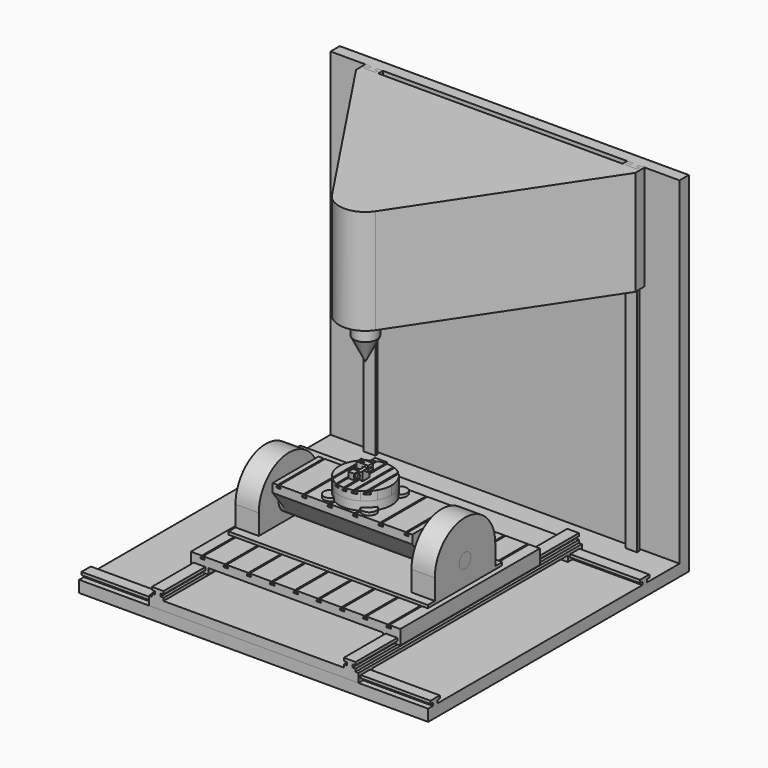
from build123d import *

# Parameters (mm, degrees)
F0_W           = 25.4
F0_H           = 12.7
F1_DEPTH       = 762
F3_DEPTH       = 457.2
F5_DEPTH       = 609.6
F7_DEPTH       = 381
F9_DEPTH       = 609.601
F9_DEPTH_BACK  = 609.601
F10_W          = 869.95
F10_H          = 12.7
F11_DEPTH      = 203.2
F14_DEPTH      = 101.6
F15_DEPTH      = 101.6
F16_R          = 31.75
F17_DEPTH      = 762.001
F17_DEPTH_BACK = 762.001
F18_R          = 31.75
F19_DEPTH      = 434.975
F19_DEPTH_BACK = 434.975
F20_DEPTH      = 333.375
F20_DEPTH_BACK = 333.375
F18_W          = 249.8384077759
F18_H          = 38.1
F21_DEPTH      = 304.8
F23_DEPTH      = 609.601
F23_DEPTH_BACK = 609.601
F25_DEPTH      = 12.7
F26_DEPTH      = 38.1
F27_DEPTH      = 38.1
F29_DEPTH      = 609.601
F29_DEPTH_BACK = 609.601
F30_DEPTH      = 152.4
F31_W          = 1524
F31_H          = 1524
F32_DEPTH      = 50.8
F34_DEPTH      = 1473.2
F36_DEPTH      = 457.2
F38_DEPTH      = 457.2
F39_R          = 50.8
F40_DEPTH      = 76.2
F44_DEPTH      = 38.1
F45_R          = 4.7625
F46_DEPTH      = 101.6
F47_W          = 19.05
F47_H          = 25.4
F48_DEPTH      = 25.4
F50_DEPTH      = 844.551
F51_R          = 4.7625
F52_DEPTH      = 101.6
F53_W          = 20.7483425409
F53_H          = 29.6389577031
F54_DEPTH      = 1035.051
F55_W          = 25.4
F55_H          = 25.4
F55_R          = 4.7625
F56_DEPTH      = 25.4
F57_R          = 7.9375
F58_DEPTH      = 9.525
F60_DEPTH      = 488.951


with BuildPart() as f1:
    # F0 (on Right) → F1 (new body, symmetric)
    with BuildSketch(Plane.YZ):
        Polygon((-558.8, -12.7), (-584.2, -12.7), (-609.6, -12.7), (-609.6, -63.5), (609.6, -63.5), (609.6, -12.7), (584.2, -12.7), (558.8, -12.7), align=None)
        Polygon((-596.9, 12.7), (-596.9, 0), (-584.2, 0), (-558.8, 0), (-546.1, 0), (-546.1, 12.7), align=None)
        with Locations((571.5, -6.35)):
            Rectangle(F0_W, F0_H)
        Polygon((546.1, 0), (558.8, 0), (584.2, 0), (596.9, 0), (596.9, 12.7), (546.1, 12.7), align=None)
        with Locations((-571.5, -6.35)):
            Rectangle(F0_W, F0_H)
    extrude(amount=F1_DEPTH, both=True)

    # F30 (add): a face of the model
    f30_faces = [f1.faces().sort_by_distance(p)[0] for p in [
        (0, 609.6, -38.1),
    ]]
    extrude(f30_faces, amount=F30_DEPTH)

    # F31 (on face) → F32 (join)
    with BuildSketch(Plane(origin=(0, 762, 0), x_dir=(-1, 0, 0), z_dir=(0, 1, 0))):
        with Locations((0, 698.5)):
            Rectangle(F31_W, F31_H)
    extrude(amount=F32_DEPTH)

    # F33 (on face) → F34 (join, through all)
    with BuildSketch(Plane.XY.offset(1460.5)):
        Polygon((584.2, 749.3), (584.2, 762), (558.8, 762), (558.8, 749.3), (546.1, 749.3), (546.1, 736.6), (596.9, 736.6), (596.9, 749.3), align=None)
        Polygon((-584.2, 762), (-584.2, 749.3), (-596.9, 749.3), (-596.9, 736.6), (-546.1, 736.6), (-546.1, 749.3), (-558.8, 749.3), (-558.8, 762), align=None)
    extrude(amount=-F34_DEPTH)


with BuildPart() as f3:
    # F2 (on Right) → F3 (new body, symmetric)
    with BuildSketch(Plane.YZ):
        Polygon((-609.6, 25.4), (-609.6, -12.7), (-584.2, -12.7), (-584.2, 0), (-596.9, 0), (-596.9, 12.7), (-546.1, 12.7), (-546.1, 0), (-558.8, 0), (-558.8, -12.7), (-533.4, -12.7), (-533.4, 12.7), (533.4, 12.7), (533.4, -12.7), (558.8, -12.7), (558.8, 0), (546.1, 0), (546.1, 12.7), (596.9, 12.7), (596.9, 0), (584.2, 0), (584.2, -12.7), (609.6, -12.7), (609.6, 25.4), align=None)
    extrude(amount=F3_DEPTH, both=True)

    # F4 (on Front) → F5 (join, symmetric)
    with BuildSketch(Plane.XZ):
        Polygon((-444.5, 38.1), (-444.5, 25.4), (-393.7, 25.4), (-393.7, 38.1), (-406.4, 38.1), (-406.4, 50.8), (-393.7, 50.8), (-393.7, 63.5), (-444.5, 63.5), (-444.5, 50.8), (-431.8, 50.8), (-431.8, 38.1), align=None)
        Polygon((393.7, 63.5), (393.7, 50.8), (406.4, 50.8), (406.4, 38.1), (393.7, 38.1), (393.7, 25.4), (444.5, 25.4), (444.5, 38.1), (431.8, 38.1), (431.8, 50.8), (444.5, 50.8), (444.5, 63.5), align=None)
    extrude(amount=F5_DEPTH, both=True)


with BuildPart() as f7:
    # F6 (on Front) → F7 (new body, symmetric)
    with BuildSketch(Plane.XZ):
        Polygon((-457.2, 38.1), (-431.8, 38.1), (-431.8, 50.8), (-444.5, 50.8), (-444.5, 63.5), (-393.7, 63.5), (-393.7, 50.8), (-406.4, 50.8), (-406.4, 38.1), (-381, 38.1), (-381, 63.5), (381, 63.5), (381, 38.1), (406.4, 38.1), (406.4, 50.8), (393.7, 50.8), (393.7, 63.5), (444.5, 63.5), (444.5, 50.8), (431.8, 50.8), (431.8, 38.1), (457.2, 38.1), (457.2, 101.6), (-457.2, 101.6), align=None)
    extrude(amount=F7_DEPTH, both=True)

    # F8 (on Front) → F9 (cut, two sides)
    with BuildSketch(Plane.XZ) as f9_sk:
        Polygon((-403.225, 101.6), (-409.575, 101.6), (-409.575, 95.25), (-415.925, 95.25), (-415.925, 88.9), (-396.875, 88.9), (-396.875, 95.25), (-403.225, 95.25), align=None)
        Polygon((-295.275, 95.25), (-301.625, 95.25), (-301.625, 101.6), (-307.975, 101.6), (-307.975, 95.25), (-314.325, 95.25), (-314.325, 88.9), (-295.275, 88.9), align=None)
        Polygon((-193.675, 95.25), (-200.025, 95.25), (-200.025, 101.6), (-206.375, 101.6), (-206.375, 95.25), (-212.725, 95.25), (-212.725, 88.9), (-193.675, 88.9), align=None)
        Polygon((-92.075, 95.25), (-98.425, 95.25), (-98.425, 101.6), (-104.775, 101.6), (-104.775, 95.25), (-111.125, 95.25), (-111.125, 88.9), (-92.075, 88.9), align=None)
        Polygon((9.525, 95.25), (3.175, 95.25), (3.175, 101.6), (-3.175, 101.6), (-3.175, 95.25), (-9.525, 95.25), (-9.525, 88.9), (9.525, 88.9), align=None)
        Polygon((111.125, 95.25), (104.775, 95.25), (104.775, 101.6), (98.425, 101.6), (98.425, 95.25), (92.075, 95.25), (92.075, 88.9), (111.125, 88.9), align=None)
        Polygon((212.725, 95.25), (206.375, 95.25), (206.375, 101.6), (200.025, 101.6), (200.025, 95.25), (193.675, 95.25), (193.675, 88.9), (212.725, 88.9), align=None)
        Polygon((314.325, 95.25), (307.975, 95.25), (307.975, 101.6), (301.625, 101.6), (301.625, 95.25), (295.275, 95.25), (295.275, 88.9), (314.325, 88.9), align=None)
        Polygon((415.925, 95.25), (409.575, 95.25), (409.575, 101.6), (403.225, 101.6), (403.225, 95.25), (396.875, 95.25), (396.875, 88.9), (415.925, 88.9), align=None)
    extrude(amount=-F9_DEPTH, mode=Mode.SUBTRACT)
    extrude(f9_sk.sketch, amount=F9_DEPTH_BACK, mode=Mode.SUBTRACT)


with BuildPart() as f11:
    # F10 (on Front) → F11 (new body, symmetric)
    with BuildSketch(Plane.XZ):
        with Locations((0, 107.95)):
            Rectangle(F10_W, F10_H)
    extrude(amount=F11_DEPTH, both=True)

    # F13 (on face) → F14 (join)
    with BuildSketch(Plane.YZ.offset(434.975)):
        with BuildLine():
            ThreePointArc((165.1, 203.2), (0, 368.3), (-165.1, 203.2))
            Line((-165.1, 203.2), (-165.1, 114.3))
            Line((-165.1, 114.3), (165.1, 114.3))
            Line((165.1, 114.3), (165.1, 203.2))
        make_face()
    extrude(amount=-F14_DEPTH)

    # F12 (on face) → F15 (join)
    with BuildSketch(Plane(origin=(-434.975, 0, 0), x_dir=(0, -1, 0), z_dir=(-1, 0, 0))):
        with BuildLine():
            Line((-165.1, 203.2), (-165.1, 114.3))
            Line((-165.1, 114.3), (165.1, 114.3))
            Line((165.1, 114.3), (165.1, 203.2))
            ThreePointArc((165.1, 203.2), (0, 368.3), (-165.1, 203.2))
        make_face()
    extrude(amount=-F15_DEPTH)

    # F16 (on Right) → F17 (cut, two sides)
    with BuildSketch(Plane.YZ) as f17_sk:
        with Locations((0, 203.2)):
            Circle(F16_R)
    extrude(amount=-F17_DEPTH, mode=Mode.SUBTRACT)
    extrude(f17_sk.sketch, amount=F17_DEPTH_BACK, mode=Mode.SUBTRACT)


with BuildPart() as f19:
    # F18 (on Right) → F19 (new body, two sides)
    with BuildSketch(Plane.YZ) as f19_sk:
        with Locations((0, 203.2)):
            Circle(F18_R)
    extrude(amount=-F19_DEPTH)
    extrude(f19_sk.sketch, amount=F19_DEPTH_BACK)

    # F18 (on Right) → F20 (join, two sides)
    with BuildSketch(Plane.YZ) as f20_sk:
        with BuildLine():
            ThreePointArc((-45.4898926883, 168.6053159689), (0, 146.05), (45.4898926883, 168.6053159689))
            ThreePointArc((45.4898926883, 168.6053159689), (54.1565779344, 184.946573844), (57.15, 203.2))
            ThreePointArc((57.15, 203.2), (-18.253426156, 257.3565779344), (-45.4898926883, 168.6053159689))
        make_face()
        with Locations((0, 203.2)):
            Circle(F18_R, mode=Mode.SUBTRACT)
    extrude(amount=F20_DEPTH)
    extrude(f20_sk.sketch, amount=-F20_DEPTH_BACK)

    # F18 (on Right) → F21 (join, symmetric)
    with BuildSketch(Plane.YZ):
        with BuildLine():
            Line((45.4898926883, 168.6053159689), (124.919203888, 273.05))
            Line((124.919203888, 273.05), (-124.919203888, 273.05))
            Line((-124.919203888, 273.05), (-45.4898926883, 168.6053159689))
            ThreePointArc((-45.4898926883, 168.6053159689), (-18.253426156, 257.3565779344), (57.15, 203.2))
            ThreePointArc((57.15, 203.2), (54.1565779344, 184.946573844), (45.4898926883, 168.6053159689))
        make_face()
        with Locations((0, 292.1)):
            Rectangle(F18_W, F18_H)
    extrude(amount=F21_DEPTH, both=True)

    # F22 (on Front) → F23 (cut, two sides)
    with BuildSketch(Plane.XZ) as f23_sk:
        Polygon((282.575, 304.8), (282.575, 311.15), (276.225, 311.15), (276.225, 304.8), (269.875, 304.8), (269.875, 298.45), (288.925, 298.45), (288.925, 304.8), align=None)
        Polygon((158.115, 304.8), (158.115, 298.45), (177.165, 298.45), (177.165, 304.8), (170.815, 304.8), (170.815, 311.15), (164.465, 311.15), (164.465, 304.8), align=None)
        Polygon((46.355, 304.8), (46.355, 298.45), (65.405, 298.45), (65.405, 304.8), (59.055, 304.8), (59.055, 311.15), (52.705, 311.15), (52.705, 304.8), align=None)
        Polygon((-65.405, 304.8), (-65.405, 298.45), (-46.355, 298.45), (-46.355, 304.8), (-52.705, 304.8), (-52.705, 311.15), (-59.055, 311.15), (-59.055, 304.8), align=None)
        Polygon((-177.165, 304.8), (-177.165, 298.45), (-158.115, 298.45), (-158.115, 304.8), (-164.465, 304.8), (-164.465, 311.15), (-170.815, 311.15), (-170.815, 304.8), align=None)
        Polygon((-288.925, 304.8), (-288.925, 298.45), (-269.875, 298.45), (-269.875, 304.8), (-276.225, 304.8), (-276.225, 311.15), (-282.575, 311.15), (-282.575, 304.8), align=None)
    extrude(amount=-F23_DEPTH, mode=Mode.SUBTRACT)
    extrude(f23_sk.sketch, amount=F23_DEPTH_BACK, mode=Mode.SUBTRACT)


with BuildPart() as f25:
    # F24 (on face) → F25 (new body)
    with BuildSketch(Plane.XY.offset(311.15)):
        with BuildLine():
            ThreePointArc((98.9867036526, -57.15), (110.4053219448, -29.5830168552), (114.3, 0))
            ThreePointArc((114.3, 0), (110.4053219448, 29.5830168552), (98.9867036526, 57.15))
            ThreePointArc((98.9867036526, 57.15), (80.8223050896, 80.8223050896), (57.15, 98.9867036526))
            ThreePointArc((57.15, 98.9867036526), (0, 114.3), (-57.15, 98.9867036526))
            ThreePointArc((-57.15, 98.9867036526), (-80.8223050896, 80.8223050896), (-98.9867036526, 57.15))
            ThreePointArc((-98.9867036526, 57.15), (-114.3, 0), (-98.9867036526, -57.15))
            ThreePointArc((-98.9867036526, -57.15), (-80.8223050896, -80.8223050896), (-57.15, -98.9867036526))
            ThreePointArc((-57.15, -98.9867036526), (0, -114.3), (57.15, -98.9867036526))
            ThreePointArc((57.15, -98.9867036526), (80.8223050896, -80.8223050896), (98.9867036526, -57.15))
        make_face()
        with BuildLine():
            ThreePointArc((57.15, 98.9867036526), (80.8223050896, 80.8223050896), (98.9867036526, 57.15))
            ThreePointArc((98.9867036526, 57.15), (105.3296786843, 105.3296786843), (57.15, 98.9867036526))
        make_face()
        with BuildLine():
            ThreePointArc((57.15, -98.9867036526), (105.3296786843, -105.3296786843), (98.9867036526, -57.15))
            ThreePointArc((98.9867036526, -57.15), (80.8223050896, -80.8223050896), (57.15, -98.9867036526))
        make_face()
        with BuildLine():
            ThreePointArc((-98.9867036526, 57.15), (-80.8223050896, 80.8223050896), (-57.15, 98.9867036526))
            ThreePointArc((-57.15, 98.9867036526), (-105.3296786843, 105.3296786843), (-98.9867036526, 57.15))
        make_face()
        with BuildLine():
            ThreePointArc((-98.9867036526, -57.15), (-105.3296786843, -105.3296786843), (-57.15, -98.9867036526))
            ThreePointArc((-57.15, -98.9867036526), (-80.8223050896, -80.8223050896), (-98.9867036526, -57.15))
        make_face()
    extrude(amount=F25_DEPTH)

    # F24 (on face) → F26 (join)
    with BuildSketch(Plane.XY.offset(311.15)):
        with BuildLine():
            ThreePointArc((98.9867036526, -57.15), (110.4053219448, -29.5830168552), (114.3, 0))
            ThreePointArc((114.3, 0), (110.4053219448, 29.5830168552), (98.9867036526, 57.15))
            ThreePointArc((98.9867036526, 57.15), (80.8223050896, 80.8223050896), (57.15, 98.9867036526))
            ThreePointArc((57.15, 98.9867036526), (0, 114.3), (-57.15, 98.9867036526))
            ThreePointArc((-57.15, 98.9867036526), (-58.1052206891, 98.4290268603), (-59.055, 97.8621324875))
            Line((-59.055, 97.8621324875), (-59.055, -97.8621324875))
            ThreePointArc((-59.055, -97.8621324875), (-58.1052206891, -98.4290268603), (-57.15, -98.9867036526))
            ThreePointArc((-57.15, -98.9867036526), (0, -114.3), (57.15, -98.9867036526))
            ThreePointArc((57.15, -98.9867036526), (80.8223050896, -80.8223050896), (98.9867036526, -57.15))
        make_face()
        with BuildLine():
            Line((-59.055, -97.8621324875), (-59.055, 97.8621324875))
            ThreePointArc((-59.055, 97.8621324875), (-81.6006400482, 80.0364013667), (-98.9867036526, 57.15))
            ThreePointArc((-98.9867036526, 57.15), (-114.3, 0), (-98.9867036526, -57.15))
            ThreePointArc((-98.9867036526, -57.15), (-81.6006400482, -80.0364013667), (-59.055, -97.8621324875))
        make_face()
    extrude(amount=F26_DEPTH)


with BuildPart() as f27:
    # F27 (new): a face of the model
    f27_faces = [f25.part.faces().sort_by_distance(p)[0] for p in [
        (0, 0, 349.25),
    ]]
    extrude(f27_faces, amount=F27_DEPTH)

    # F28 (on Front) → F29 (cut, two sides)
    with BuildSketch(Plane.XZ) as f29_sk:
        Polygon((79.375, 381), (79.375, 387.35), (73.025, 387.35), (73.025, 381), (66.675, 381), (66.675, 374.65), (85.725, 374.65), (85.725, 381), align=None)
        Polygon((41.275, 381), (41.275, 387.35), (34.925, 387.35), (34.925, 381), (28.575, 381), (28.575, 374.65), (47.625, 374.65), (47.625, 381), align=None)
        Polygon((3.175, 381), (3.175, 387.35), (-3.175, 387.35), (-3.175, 381), (-9.525, 381), (-9.525, 374.65), (9.525, 374.65), (9.525, 381), align=None)
        Polygon((-34.925, 381), (-34.925, 387.35), (-41.275, 387.35), (-41.275, 381), (-47.625, 381), (-47.625, 374.65), (-28.575, 374.65), (-28.575, 381), align=None)
        Polygon((-73.025, 381), (-73.025, 387.35), (-79.375, 387.35), (-79.375, 381), (-85.725, 381), (-85.725, 374.65), (-66.675, 374.65), (-66.675, 381), align=None)
    extrude(amount=-F29_DEPTH, mode=Mode.SUBTRACT)
    extrude(f29_sk.sketch, amount=F29_DEPTH_BACK, mode=Mode.SUBTRACT)


with BuildPart() as f36:
    # F35 (on face) → F36 (new body)
    with BuildSketch(Plane.XY.offset(1460.5)):
        Polygon((609.6, 762), (584.2, 762), (584.2, 749.3), (596.9, 749.3), (596.9, 736.6), (546.1, 736.6), (546.1, 749.3), (558.8, 749.3), (558.8, 762), (533.4, 762), (533.4, 736.6), (-533.4, 736.6), (-533.4, 762), (-558.8, 762), (-558.8, 749.3), (-546.1, 749.3), (-546.1, 736.6), (-596.9, 736.6), (-596.9, 749.3), (-584.2, 749.3), (-584.2, 762), (-609.6, 762), (-609.6, 711.2), (609.6, 711.2), align=None)
    extrude(amount=-F36_DEPTH)

    # F37 (on face) → F38 (join, through all)
    with BuildSketch(Plane.XY.offset(1460.5)):
        with BuildLine():
            Line((-609.6, 711.2), (-95.2112843784, -63.2400294672))
            ThreePointArc((-95.2112843784, -63.2400294672), (0, -114.3), (95.2112843784, -63.2400294672))
            Line((95.2112843784, -63.2400294672), (609.6, 711.2))
            Line((609.6, 711.2), (-609.6, 711.2))
        make_face()
    extrude(amount=-F38_DEPTH)

    # F39 (on face) → F40 (join)
    with BuildSketch(Plane(origin=(0, 0, 1003.3), x_dir=(1, 0, 0), z_dir=(0, 0, -1))):
        Circle(F39_R)
    extrude(amount=F40_DEPTH)

    # F41 (on Right) → F42 (revolve)
    with BuildSketch(Plane.YZ):
        Polygon((0, 825.5), (0, 927.1), (-50.8, 927.1), align=None)
    revolve(axis=Axis((0, 0, 876.3), (0, 0, -1)))


with BuildPart() as f44:
    # F43 (on Front) → F44 (new body)
    with BuildSketch(Plane.XZ):
        Polygon((-19.6643165916, 425.45), (-19.6643165916, 387.35), (-13.3143165916, 387.35), (-6.9643165916, 393.7), (5.7356834084, 393.7), (12.0856834084, 387.35), (18.4356834084, 387.35), (18.4356834084, 425.45), align=None)
    extrude(amount=F44_DEPTH)

    # F45 (on face) → F46 (join)
    with BuildSketch(Plane.XY.offset(425.45)):
        with Locations((-0.6143165916, -19.05)):
            Circle(F45_R)
    extrude(amount=F46_DEPTH)

    # F53 (on face) → F54 (cut, through all)
    with BuildSketch(Plane.XY.offset(425.45)):
        with Locations((-0.6143165916, -19.05)):
            Rectangle(F53_W, F53_H)
    extrude(amount=F54_DEPTH, mode=Mode.SUBTRACT)

    # F59 (on face) → F60 (cut, through all)
    with BuildSketch(Plane.XY.offset(425.45)):
        Polygon((5.7356834084, -6.35), (12.0856834084, 0), (-13.3143165916, 0), (-6.9643165916, -6.35), align=None)
    extrude(amount=-F60_DEPTH, mode=Mode.SUBTRACT)


with BuildPart() as f48:
    # F47 (on face) → F48 (new body)
    with BuildSketch(Plane.XY.offset(425.45)):
        with BuildLine():
            Line((18.4356834084, -6.35), (-13.3143165916, -6.35))
            Line((-13.3143165916, -6.35), (-13.3143165916, -17.4625))
            Line((-13.3143165916, -17.4625), (-5.1044446522, -17.4625))
            ThreePointArc((-5.1044446522, -17.4625), (-0.6143165916, -14.2875), (3.8758114689, -17.4625))
            Line((3.8758114689, -17.4625), (12.0856834084, -17.4625))
            Line((12.0856834084, -17.4625), (12.0856834084, -20.6375))
            Line((12.0856834084, -20.6375), (3.8758114689, -20.6375))
            ThreePointArc((3.8758114689, -20.6375), (-0.6143165916, -23.8125), (-5.1044446522, -20.6375))
            Line((-5.1044446522, -20.6375), (-13.3143165916, -20.6375))
            Line((-13.3143165916, -20.6375), (-13.3143165916, -31.75))
            Line((-13.3143165916, -31.75), (18.4356834084, -31.75))
            Line((18.4356834084, -31.75), (18.4356834084, -6.35))
        make_face()
        with Locations((27.9606834084, -19.05)):
            Rectangle(F47_W, F47_H)
    extrude(amount=F48_DEPTH)

    # F49 (on face) → F50 (cut, through all)
    with BuildSketch(Plane.XZ.offset(31.75)):
        with BuildLine():
            Line((20.2955553478, 439.7375), (29.2758114689, 439.7375))
            ThreePointArc((29.2758114689, 439.7375), (24.7856834084, 442.9125), (20.2955553478, 439.7375))
        make_face()
        with BuildLine():
            ThreePointArc((20.2955553478, 436.5625), (24.7856834084, 433.3875), (29.2758114689, 436.5625))
            Line((29.2758114689, 436.5625), (20.2955553478, 436.5625))
        make_face()
        with BuildLine():
            ThreePointArc((29.2758114689, 436.5625), (29.4795965487, 437.3446518263), (29.5481834084, 438.15))
            ThreePointArc((29.5481834084, 438.15), (29.4795965487, 438.9553481737), (29.2758114689, 439.7375))
            Line((29.2758114689, 439.7375), (20.2955553478, 439.7375))
            ThreePointArc((20.2955553478, 439.7375), (20.0231834084, 438.15), (20.2955553478, 436.5625))
            Line((20.2955553478, 436.5625), (29.2758114689, 436.5625))
        make_face()
        with BuildLine():
            ThreePointArc((20.2955553478, 436.5625), (20.0231834084, 438.15), (20.2955553478, 439.7375))
            Line((20.2955553478, 439.7375), (12.0856834084, 439.7375))
            Line((12.0856834084, 439.7375), (12.0856834084, 436.5625))
            Line((12.0856834084, 436.5625), (20.2955553478, 436.5625))
        make_face()
        with BuildLine():
            ThreePointArc((29.2758114689, 439.7375), (29.4795965487, 438.9553481737), (29.5481834084, 438.15))
            ThreePointArc((29.5481834084, 438.15), (29.4795965487, 437.3446518263), (29.2758114689, 436.5625))
            Line((29.2758114689, 436.5625), (37.4856834084, 436.5625))
            Line((37.4856834084, 436.5625), (37.4856834084, 439.7375))
            Line((37.4856834084, 439.7375), (29.2758114689, 439.7375))
        make_face()
    extrude(amount=-F50_DEPTH, mode=Mode.SUBTRACT)


with BuildPart() as f52:
    # F51 (on face) → F52 (new body)
    with BuildSketch(Plane(origin=(0, -6.35, 0), x_dir=(-1, 0, 0), z_dir=(0, 1, 0))):
        with Locations((-24.7856834084, 438.15)):
            Circle(F51_R)
    extrude(amount=-F52_DEPTH)


with BuildPart() as f56:
    # F55 (on face) → F56 (new body)
    with BuildSketch(Plane.XZ.offset(107.95)):
        with Locations((24.7856834084, 438.15)):
            Rectangle(F55_W, F55_H)
        with Locations((24.7856834084, 438.15)):
            Circle(F55_R, mode=Mode.SUBTRACT)
    extrude(amount=-F56_DEPTH)

    # F57 (on face) → F58 (join)
    with BuildSketch(Plane.YZ.offset(37.4856834084)):
        with Locations((-95.25, 438.15)):
            Circle(F57_R)
    extrude(amount=F58_DEPTH)


solid = Compound([f1.part, f3.part, f7.part, f11.part, f19.part, f25.part, f27.part, f36.part, f44.part, f48.part, f52.part, f56.part])
